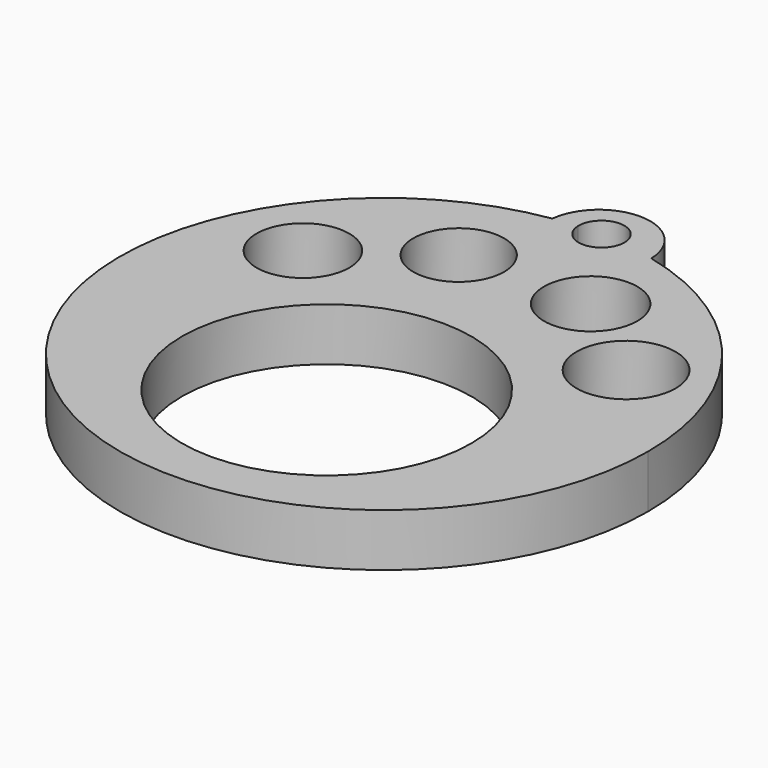
from build123d import *

# Parameters (mm, degrees)
F0_R     = 13.705866293
F0_R_2   = 4.3874864706
F0_R_3   = 4.303486485
F0_R_4   = 4.6919029461
F0_R_5   = 4.4212893062
F1_DEPTH = 5


# Not quite as in the source:
# - a feature names something its author has since deleted; it is built from what else it names


with BuildPart() as f1:
    # F0 (on Top) → F1 (new body)
    with BuildSketch(Plane.XY):
        with BuildLine():
            ThreePointArc((-21.5933528567, 15.5303339684), (-34.0411472206, -28.1567693277), (7.2290643581, -9.1757204846))
            ThreePointArc((7.2290643581, -9.1757204846), (1.8714254099, 6.2896489682), (-11.9051478269, 15.1263891627))
            ThreePointArc((-11.9051478269, 15.1263891627), (-13.4691027147, 15.4513831507), (-15.0506199283, 15.6758364569))
            ThreePointArc((-15.0506199283, 15.6758364569), (-17.255118812, 13.6982838706), (-19.3682330997, 15.77320015))
            ThreePointArc((-19.3682330997, 15.77320015), (-20.4835124203, 15.6766823614), (-21.5933528567, 15.5303339684))
        make_face()
        with Locations((-17.4914449453, -16.3063649088)):
            Circle(F0_R, mode=Mode.SUBTRACT)
        with Locations((-32.7908843756, 0)):
            Circle(F0_R_2, mode=Mode.SUBTRACT)
        with Locations((-23.3562290668, 6.6427942365)):
            Circle(F0_R_3, mode=Mode.SUBTRACT)
        with Locations((-2.1920050494, 0)):
            Circle(F0_R_4, mode=Mode.SUBTRACT)
        with Locations((-10.8616864309, 6.6427942365)):
            Circle(F0_R_5, mode=Mode.SUBTRACT)
        with BuildLine():
            ThreePointArc((-15.0506199283, 15.6758364569), (-13.4691027147, 15.4513831507), (-11.9051478269, 15.1263891627))
            ThreePointArc((-11.9051478269, 15.1263891627), (-16.560489471, 19.8555989303), (-21.5933528567, 15.5303339684))
            ThreePointArc((-21.5933528567, 15.5303339684), (-20.4835124203, 15.6766823614), (-19.3682330997, 15.77320015))
            ThreePointArc((-19.3682330997, 15.77320015), (-17.2504619715, 18.0246709507), (-15.0426456956, 15.8614274114))
            ThreePointArc((-15.0426456956, 15.8614274114), (-15.044640173, 15.768546317), (-15.0506199283, 15.6758364569))
        make_face()
    extrude(amount=F1_DEPTH)


solid = f1.part
